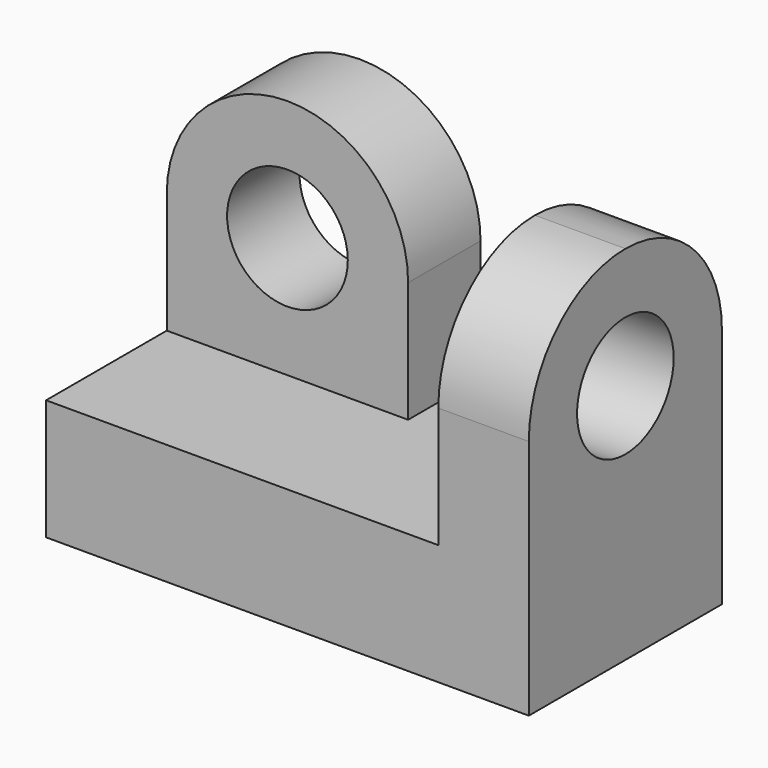
from build123d import *

# Parameters (mm, degrees)
F1_DEPTH = 40
F0_R     = 10
F2_DEPTH = 15
F3_R     = 19.99999
F4_R     = 10
F5_DEPTH = 15


# Not quite as in the source:
# - a fillet or chamfer is up to 0.001 mm smaller than in the source, because OpenCascade refuses the exact size


with BuildPart() as f1:
    # F0 (on Front) → F1 (new body)
    with BuildSketch(Plane.XZ):
        Polygon((0, 20), (0, 0), (80, 0), (80, 60), (65, 60), (65, 20), (40, 20), align=None)
    extrude(amount=F1_DEPTH)

    # F0 (on Front) → F2 (join)
    with BuildSketch(Plane.XZ):
        with BuildLine():
            Line((0, 40), (0, 20))
            Line((0, 20), (40, 20))
            Line((40, 20), (40, 40))
            ThreePointArc((40, 40), (20, 60), (0, 40))
        make_face()
        with Locations((20, 40)):
            Circle(F0_R, mode=Mode.SUBTRACT)
    extrude(amount=F2_DEPTH)

    # F3 (radius 20 in the source; OpenCascade refuses exactly that, so slightly less here)
    f3_edges = [f1.edges().sort_by_distance(p)[0] for p in [
        (72.5, -40, 60),
        (72.5, 0, 60),
    ]]
    fillet(f3_edges, radius=F3_R)

    # F4 (on face) → F5 (cut, through all)
    with BuildSketch(Plane.YZ.offset(80)):
        with Locations((-20, 40)):
            Circle(F4_R)
    extrude(amount=-F5_DEPTH, mode=Mode.SUBTRACT)


solid = f1.part
